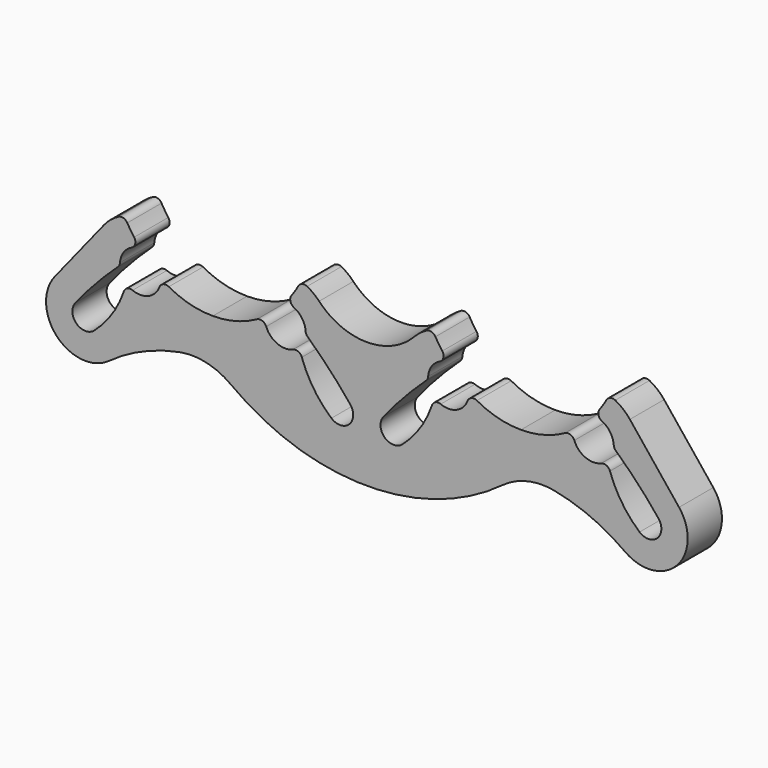
from build123d import *

# Parameters (mm, degrees)
F2_DEPTH = 1.625
F3_R     = 0.5
F7_R     = 5
F9_DEPTH = 1.625
F10_R    = 5


with BuildPart() as f2:
    # F1 (on Front) → F2 (new body, symmetric)
    with BuildSketch(Plane.XZ):
        with BuildLine():
            ThreePointArc((0, -6.875), (-2.0724417463, -6.5551971906), (-3.9520768911, -5.6255411515))
            ThreePointArc((-3.9520768911, -5.6255411515), (-4.8570002775, -7.1160909953), (-6.5757097792, -6.8217054979))
            ThreePointArc((-6.5757097792, -6.8217054979), (-7.4894639741, -8.9857797177), (-9.0066893746, -10.7791539234))
            ThreePointArc((-9.0066893746, -10.7791539234), (-10.3561219729, -10.7473840389), (-10.4445927673, -9.400479966))
            ThreePointArc((-10.4445927673, -9.400479966), (-8.8177667586, -7.5260240462), (-7.0479231089, -5.7859661986))
            ThreePointArc((-7.0479231089, -5.7859661986), (-6.6159518229, -4.6300438958), (-5.4766665535, -4.1559293139))
            ThreePointArc((-5.4766665535, -4.1559293139), (-6.1554446566, -3.3057655277), (-6.7033968415, -2.3659428957))
            ThreePointArc((-6.7033968415, -2.3659428957), (-7.5646836603, -2.8179203379), (-8.2709699391, -3.4866940551))
            Line((-8.2709699391, -3.4866940551), (-12.0057025921, -8.1503055323))
            ThreePointArc((-12.0057025921, -8.1503055323), (-11.8324993376, -12.098674705), (-7.8959026306, -12.4491384793))
            ThreePointArc((-7.8959026306, -12.4491384793), (-4.1524531082, -10.534781214), (0, -9.875))
            Line((0, -9.875), (0, -6.875))
        make_face()
    extrude(amount=F2_DEPTH, both=True)

    # F3
    f3_edges = [f2.edges().sort_by_distance(p)[0] for p in [
        (-3.952077, 0, -5.625541),
        (-7.047923, 0, -5.785966),
        (-6.703397, 0, -2.365943),
        (-5.476667, 0, -4.155929),
        (-6.57571, 0, -6.821705),
    ]]
    fillet(f3_edges, radius=F3_R)

    # F4: F2 across plane


with BuildPart() as f2_1:
    add(f2.part)
    add(f2.part.mirror(Plane.YZ))


with BuildPart() as f5_1:
    # F5: copy of F2
    add(f2_1.part.moved(Location((23.4, 0, 0))))


with BuildPart() as f2_2:
    add(f2_1.part)

    # F6: union F5_1
    add(f5_1.part)

    # F7
    f7_edges = [f2_2.edges().sort_by_distance(p)[0] for p in [
        (11.7, 0, -7.768571),
        (11.7, 0, -12.228941),
    ]]
    fillet(f7_edges, radius=F7_R)

    # F8 (on Front) → F9 (join, symmetric)
    with BuildSketch(Plane.XZ):
        with BuildLine():
            ThreePointArc((7.8959026306, -12.4491384793), (4.1524531082, -10.534781214), (0, -9.875))
            ThreePointArc((0, -9.875), (11.7, -14.4267892403), (23.4, -9.875))
            ThreePointArc((23.4, -9.875), (19.2475468918, -10.534781214), (15.5040973694, -12.4491384793))
            ThreePointArc((15.5040973694, -12.4491384793), (14.2921704484, -12.9735550261), (12.9724763407, -12.9267892403))
            ThreePointArc((12.9724763407, -12.9267892403), (11.7, -12.762159336), (10.4275236593, -12.9267892403))
            ThreePointArc((10.4275236593, -12.9267892403), (9.1078295516, -12.9735550261), (7.8959026306, -12.4491384793))
        make_face()
    extrude(amount=F9_DEPTH, both=True)

    # F10
    f10_edges = [f2_2.edges().sort_by_distance(p)[0] for p in [
        (23.4, 0, -9.875),
        (0, 0, -9.875),
    ]]
    fillet(f10_edges, radius=F10_R)


solid = f2_2.part
